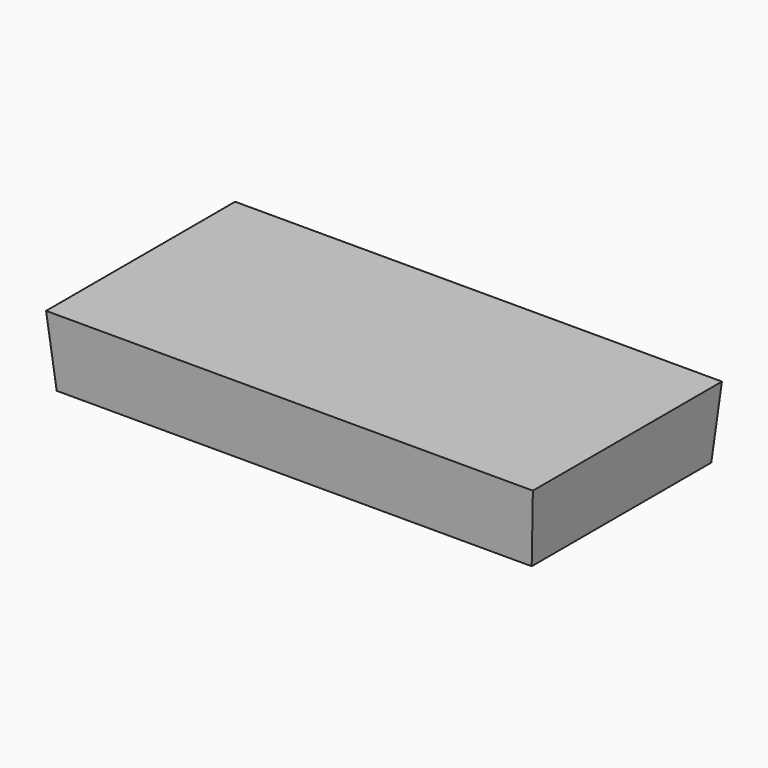
from build123d import *

# Parameters (mm, degrees)
F0_W     = 82.4
F0_H     = 40
F1_DEPTH = 12
F2_SIZE2 = 11.99999
F2_SIZE  = 0.99999


# Not quite as in the source:
# - a fillet or chamfer is up to 0.001 mm smaller than in the source, because OpenCascade refuses the exact size


with BuildPart() as f1:
    # F0 (on Top) → F1 (new body)
    with BuildSketch(Plane.XY):
        Rectangle(F0_W, F0_H)
    extrude(amount=F1_DEPTH)

    # F2 (size 1 and 12 in the source; OpenCascade refuses exactly that, so slightly less here)
    f2_edges = [f1.edges().sort_by_distance(p)[0] for p in [
        (0, -20, 0),
        (41.2, 0, 0),
        (0, 20, 0),
        (-41.2, 0, 0),
    ]]
    f2_side = f1.faces().sort_by_distance((0, 0, 0))[0]
    chamfer(f2_edges, length=F2_SIZE, length2=F2_SIZE2, reference=f2_side)


solid = f1.part
